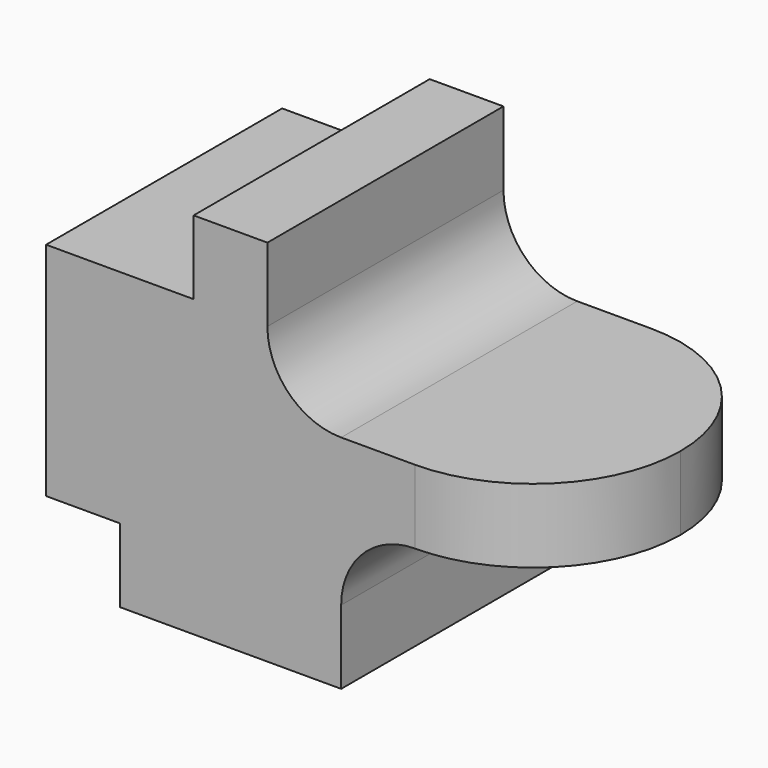
from build123d import *

# Parameters (mm, degrees)
F1_DEPTH = 20
F2_R     = 19.99999


# Not quite as in the source:
# - a fillet or chamfer is up to 0.001 mm smaller than in the source, because OpenCascade refuses the exact size


with BuildPart() as f1:
    # F0 (on Front) → F1 (new body, symmetric)
    with BuildSketch(Plane.XZ):
        with BuildLine():
            Line((0, 30), (0, 0))
            Line((0, 0), (10, 0))
            Line((10, 0), (10, -10))
            Line((10, -10), (40, -10))
            Line((40, -10), (40, 0))
            ThreePointArc((40, 0), (42.9289321881, 7.0710678119), (50, 10))
            Line((50, 10), (70, 10))
            Line((70, 10), (70, 20))
            Line((70, 20), (40, 20))
            ThreePointArc((40, 20), (32.9289321881, 22.9289321881), (30, 30))
            Line((30, 30), (30, 40))
            Line((30, 40), (20, 40))
            Line((20, 40), (20, 30))
            Line((20, 30), (0, 30))
        make_face()
    extrude(amount=F1_DEPTH, both=True)

    # F2 (radius 20 in the source; OpenCascade refuses exactly that, so slightly less here)
    f2_edges = [f1.edges().sort_by_distance(p)[0] for p in [
        (70, -20, 15),
        (70, 20, 15),
    ]]
    fillet(f2_edges, radius=F2_R)


solid = f1.part
